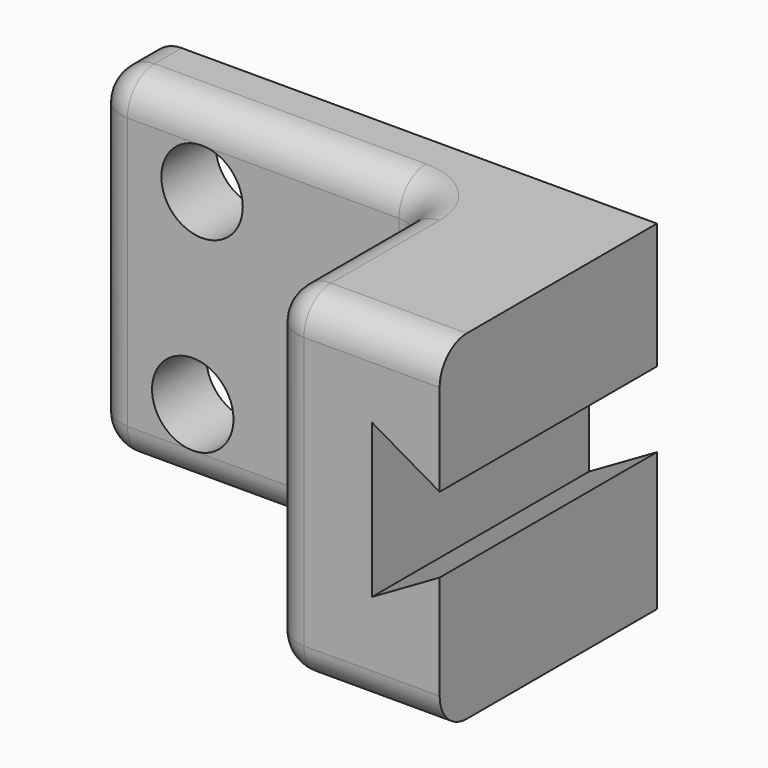
from build123d import *

# Parameters (mm, degrees)
F0_W     = 75
F0_H     = 50
F0_R     = 6
F1_DEPTH = 10
F2_W     = 25
F2_H     = 50
F3_DEPTH = 30
F5_DEPTH = 40.001
F6_R     = 5
F7_R     = 4.99999


# Not quite as in the source:
# - a fillet or chamfer is up to 0.001 mm smaller than in the source, because OpenCascade refuses the exact size


with BuildPart() as f1:
    # F0 (on Front) → F1 (new body)
    with BuildSketch(Plane.XZ):
        with Locations((-12.5, 0)):
            Rectangle(F0_W, F0_H)
        with Locations((-35.368822515, -14)):
            Circle(F0_R, mode=Mode.SUBTRACT)
        with Locations((-14, 0)):
            Circle(F0_R, mode=Mode.SUBTRACT)
        with Locations((-34, 14)):
            Circle(F0_R, mode=Mode.SUBTRACT)
    extrude(amount=F1_DEPTH)

    # F2 (on face) → F3 (join)
    with BuildSketch(Plane.XZ.offset(10)):
        with Locations((12.5, 0)):
            Rectangle(F2_W, F2_H)
    extrude(amount=F3_DEPTH)

    # F4 (on face) → F5 (cut, through all)
    with BuildSketch(Plane.XZ.offset(40)):
        Polygon((25, -4.6425589255), (25, 6.4739544771), (15, 12.247457169), (15, -10.4160616174), align=None)
    extrude(amount=-F5_DEPTH, mode=Mode.SUBTRACT)

    # F6
    f6_edges = [f1.edges().sort_by_distance(p)[0] for p in [
        (-50, -5, -25),
        (-50, -5, 25),
        (0, -10, 0),
    ]]
    fillet(f6_edges, radius=F6_R)

    # F7 (radius 5 in the source; OpenCascade refuses exactly that, so slightly less here)
    f7_edges = [f1.edges().sort_by_distance(p)[0] for p in [
        (-25, -10, -25),
        (12.5, -40, -25),
        (0, -40, 0),
        (12.5, -40, 25),
    ]]
    fillet(f7_edges, radius=F7_R)


solid = f1.part
